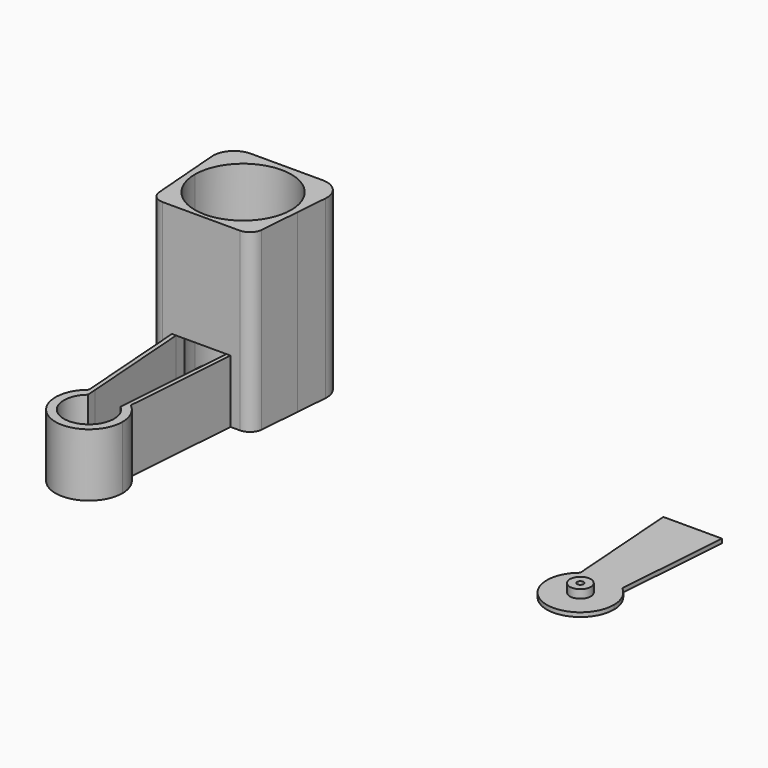
from build123d import *

# Parameters (mm, degrees)
F1_DEPTH  = 42
F2_DEPTH  = 15
F3_DEPTH  = 42
F4_DEPTH  = 15
F5_DEPTH  = 1
F0_R      = 2.5
F6_DEPTH  = 1
F0_R_2    = 1
F7_DEPTH  = 4
F8_DEPTH  = 1
F9_DEPTH  = 1
F0_R_3    = 0.75
F10_DEPTH = 3


with BuildPart() as f1:
    # F0 (on Top) → F1 (new body)
    with BuildSketch(Plane.XY):
        with BuildLine():
            Line((-12.9785589716, 24.8787840627), (-11.5, 24.8787840627))
            ThreePointArc((-11.5, 24.8787840627), (0, 36.3787840627), (11.5, 24.8787840627))
            Line((11.5, 24.8787840627), (12.9785589716, 24.8787840627))
            Line((12.9785589716, 24.8787840627), (13.5779219878, 32.533194811))
            ThreePointArc((13.5779219878, 32.533194811), (12.264120187, 36.318246043), (8.593180242, 37.923514843))
            Line((8.593180242, 37.923514843), (-8.593180242, 37.923514843))
            ThreePointArc((-8.593180242, 37.923514843), (-12.264120187, 36.318246043), (-13.5779219878, 32.533194811))
            Line((-13.5779219878, 32.533194811), (-12.9785589716, 24.8787840627))
        make_face()
        with BuildLine():
            ThreePointArc((11.5, 24.8787840627), (10.0894369384, 19.3603366119), (6.2037804754, 15.1956488363))
            Line((6.2037804754, 15.1956488363), (5.997311801, 12.3816961423))
            Line((5.997311801, 12.3816961423), (7, 12.3816961423))
            Line((7, 12.3816961423), (9.2257259033, 12.3816961423))
            ThreePointArc((9.2257259033, 12.3816961423), (11.2625646233, 13.1791321752), (12.2165709508, 15.1475041231))
            Line((12.2165709508, 15.1475041231), (12.9785589716, 24.8787840627))
            Line((12.9785589716, 24.8787840627), (11.5, 24.8787840627))
        make_face()
        with BuildLine():
            Line((-5.997311801, 12.3816961423), (-6.2037804754, 15.1956488363))
            ThreePointArc((-6.2037804754, 15.1956488363), (-10.0894369384, 19.3603366119), (-11.5, 24.8787840627))
            Line((-11.5, 24.8787840627), (-12.9785589716, 24.8787840627))
            Line((-12.9785589716, 24.8787840627), (-12.2165709508, 15.1475041231))
            ThreePointArc((-12.2165709508, 15.1475041231), (-11.2625646233, 13.1791321752), (-9.2257259033, 12.3816961423))
            Line((-9.2257259033, 12.3816961423), (-7, 12.3816961423))
            Line((-7, 12.3816961423), (-5.997311801, 12.3816961423))
        make_face()
    extrude(amount=F1_DEPTH)

    # F0 (on Top) → F2 (join)
    with BuildSketch(Plane.XY):
        with BuildLine():
            Line((-4.0454986584, -14.219481329), (-5.997311801, 12.3816961423))
            Line((-5.997311801, 12.3816961423), (-7, 12.3816961423))
            Line((-7, 12.3816961423), (-5, -14.8762179389))
            ThreePointArc((-5, -14.8762179389), (-4.5346540374, -14.5305473247), (-4.0454986584, -14.219481329))
        make_face()
        with BuildLine():
            Line((7, 12.3816961423), (5.997311801, 12.3816961423))
            Line((5.997311801, 12.3816961423), (4.0454986584, -14.219481329))
            ThreePointArc((4.0454986584, -14.219481329), (4.5346540374, -14.5305473247), (5, -14.8762179389))
            Line((5, -14.8762179389), (7, 12.3816961423))
        make_face()
        with BuildLine():
            Line((-3.8751972264, -16.5405122298), (-4.0454986584, -14.219481329))
            ThreePointArc((-4.0454986584, -14.219481329), (-4.5346540374, -14.5305473247), (-5, -14.8762179389))
            ThreePointArc((-5, -14.8762179389), (-3.4641016151, -28.3323184883), (8, -21.1212159373))
            ThreePointArc((8, -21.1212159373), (7.2111025509, -17.6571143222), (5, -14.8762179389))
            ThreePointArc((5, -14.8762179389), (4.5346540374, -14.5305473247), (4.0454986584, -14.219481329))
            Line((4.0454986584, -14.219481329), (3.8751972264, -16.5405122298))
            ThreePointArc((3.8751972264, -16.5405122298), (5.4429396175, -18.5964568754), (6, -21.1212159373))
            ThreePointArc((6, -21.1212159373), (-2.5247590619, -26.5641555548), (-3.8751972264, -16.5405122298))
        make_face()
    extrude(amount=F2_DEPTH)

    # F0 (on Top) → F3 (join)
    with BuildSketch(Plane.XY):
        with BuildLine():
            ThreePointArc((6.2037804754, 15.1956488363), (0, 13.3787840627), (-6.2037804754, 15.1956488363))
            Line((-6.2037804754, 15.1956488363), (-5.997311801, 12.3816961423))
            Line((-5.997311801, 12.3816961423), (5.997311801, 12.3816961423))
            Line((5.997311801, 12.3816961423), (6.2037804754, 15.1956488363))
        make_face()
    extrude(amount=F3_DEPTH)

    # F0 (on Top) → F4 (cut)
    with BuildSketch(Plane.XY):
        with BuildLine():
            ThreePointArc((6.2037804754, 15.1956488363), (0, 13.3787840627), (-6.2037804754, 15.1956488363))
            Line((-6.2037804754, 15.1956488363), (-5.997311801, 12.3816961423))
            Line((-5.997311801, 12.3816961423), (5.997311801, 12.3816961423))
            Line((5.997311801, 12.3816961423), (6.2037804754, 15.1956488363))
        make_face()
    extrude(amount=F4_DEPTH, mode=Mode.SUBTRACT)

    # F0 (on Top) → F5 (join)
    with BuildSketch(Plane.XY):
        with BuildLine():
            ThreePointArc((-11.5, 24.8787840627), (-10.0894369384, 19.3603366119), (-6.2037804754, 15.1956488363))
            ThreePointArc((-6.2037804754, 15.1956488363), (0, 13.3787840627), (6.2037804754, 15.1956488363))
            ThreePointArc((6.2037804754, 15.1956488363), (10.0894369384, 19.3603366119), (11.5, 24.8787840627))
            Line((11.5, 24.8787840627), (9.5, 24.8787840627))
            ThreePointArc((9.5, 24.8787840627), (0, 15.3787840627), (-9.5, 24.8787840627))
            Line((-9.5, 24.8787840627), (-11.5, 24.8787840627))
        make_face()
        with BuildLine():
            ThreePointArc((11.5, 24.8787840627), (0, 36.3787840627), (-11.5, 24.8787840627))
            Line((-11.5, 24.8787840627), (-9.5, 24.8787840627))
            ThreePointArc((-9.5, 24.8787840627), (0, 34.3787840627), (9.5, 24.8787840627))
            Line((9.5, 24.8787840627), (11.5, 24.8787840627))
        make_face()
        with BuildLine():
            Line((5.997311801, 12.3816961423), (-5.997311801, 12.3816961423))
            Line((-5.997311801, 12.3816961423), (-4.0454986584, -14.219481329))
            ThreePointArc((-4.0454986584, -14.219481329), (0, -13.1212159373), (4.0454986584, -14.219481329))
            Line((4.0454986584, -14.219481329), (5.997311801, 12.3816961423))
        make_face()
        with BuildLine():
            Line((0, 24.8787840627), (-9.5, 24.8787840627))
            ThreePointArc((-9.5, 24.8787840627), (0, 15.3787840627), (9.5, 24.8787840627))
            Line((9.5, 24.8787840627), (0, 24.8787840627))
        make_face()
        with BuildLine():
            ThreePointArc((9.5, 24.8787840627), (0, 34.3787840627), (-9.5, 24.8787840627))
            Line((-9.5, 24.8787840627), (0, 24.8787840627))
            Line((0, 24.8787840627), (9.5, 24.8787840627))
        make_face()
    extrude(amount=F5_DEPTH)

    # F0 (on Top) → F6 (join)
    with BuildSketch(Plane.XY):
        with BuildLine():
            Line((5.997311801, 12.3816961423), (-5.997311801, 12.3816961423))
            Line((-5.997311801, 12.3816961423), (-4.0454986584, -14.219481329))
            ThreePointArc((-4.0454986584, -14.219481329), (0, -13.1212159373), (4.0454986584, -14.219481329))
            Line((4.0454986584, -14.219481329), (5.997311801, 12.3816961423))
        make_face()
        with BuildLine():
            ThreePointArc((3.8751972264, -16.5405122298), (0, -15.1212159373), (-3.8751972264, -16.5405122298))
            ThreePointArc((-3.8751972264, -16.5405122298), (-2.5247590619, -26.5641555548), (6, -21.1212159373))
            ThreePointArc((6, -21.1212159373), (5.4429396175, -18.5964568754), (3.8751972264, -16.5405122298))
        make_face()
        with Locations((0, -21.1212159373)):
            Circle(F0_R, mode=Mode.SUBTRACT)
        with BuildLine():
            ThreePointArc((4.0454986584, -14.219481329), (0, -13.1212159373), (-4.0454986584, -14.219481329))
            Line((-4.0454986584, -14.219481329), (-3.8751972264, -16.5405122298))
            ThreePointArc((-3.8751972264, -16.5405122298), (0, -15.1212159373), (3.8751972264, -16.5405122298))
            Line((3.8751972264, -16.5405122298), (4.0454986584, -14.219481329))
        make_face()
        with BuildLine():
            ThreePointArc((6.2037804754, 15.1956488363), (0, 13.3787840627), (-6.2037804754, 15.1956488363))
            Line((-6.2037804754, 15.1956488363), (-5.997311801, 12.3816961423))
            Line((-5.997311801, 12.3816961423), (5.997311801, 12.3816961423))
            Line((5.997311801, 12.3816961423), (6.2037804754, 15.1956488363))
        make_face()
    extrude(amount=F6_DEPTH)

    # F0 (on Top) → F7 (join)
    with BuildSketch(Plane.XY):
        with Locations((0, -21.1212159373)):
            Circle(F0_R)
        with Locations((0, -21.1212159373)):
            Circle(F0_R_2, mode=Mode.SUBTRACT)
    extrude(amount=F7_DEPTH)

    # F0 (on Top) → F8 (join)
    with BuildSketch(Plane.XY):
        with Locations((0, -21.1212159373)):
            Circle(F0_R_2)
    extrude(amount=F8_DEPTH)


with BuildPart() as f5:
    # F0 (on Top) → F5, piece 2 (new body)
    with BuildSketch(Plane.XY):
        with BuildLine():
            Line((106.908822805, 32.923514843), (94.914199203, 32.923514843))
            Line((94.914199203, 32.923514843), (96.8660123455, 6.3223373718))
            ThreePointArc((96.8660123455, 6.3223373718), (100.911511004, 7.4206027634), (104.9570096624, 6.3223373718))
            Line((104.9570096624, 6.3223373718), (106.908822805, 32.923514843))
        make_face()
    extrude(amount=F5_DEPTH)

    # F0 (on Top) → F9 (join)
    with BuildSketch(Plane.XY):
        with BuildLine():
            Line((96.8660123455, 6.3223373718), (94.914199203, 32.923514843))
            Line((94.914199203, 32.923514843), (93.911511004, 32.923514843))
            Line((93.911511004, 32.923514843), (95.911511004, 5.6656007618))
            ThreePointArc((95.911511004, 5.6656007618), (96.3768569666, 6.011271376), (96.8660123455, 6.3223373718))
        make_face()
        with BuildLine():
            Line((107.911511004, 32.923514843), (106.908822805, 32.923514843))
            Line((106.908822805, 32.923514843), (104.9570096624, 6.3223373718))
            ThreePointArc((104.9570096624, 6.3223373718), (105.4461650413, 6.011271376), (105.911511004, 5.6656007618))
            Line((105.911511004, 5.6656007618), (107.911511004, 32.923514843))
        make_face()
        with BuildLine():
            Line((106.908822805, 32.923514843), (94.914199203, 32.923514843))
            Line((94.914199203, 32.923514843), (96.8660123455, 6.3223373718))
            ThreePointArc((96.8660123455, 6.3223373718), (100.911511004, 7.4206027634), (104.9570096624, 6.3223373718))
            Line((104.9570096624, 6.3223373718), (106.908822805, 32.923514843))
        make_face()
        with BuildLine():
            ThreePointArc((104.9570096624, 6.3223373718), (100.911511004, 7.4206027634), (96.8660123455, 6.3223373718))
            Line((96.8660123455, 6.3223373718), (97.0363137775, 4.0013064709))
            ThreePointArc((97.0363137775, 4.0013064709), (100.911511004, 5.4206027634), (104.7867082304, 4.0013064709))
            Line((104.7867082304, 4.0013064709), (104.9570096624, 6.3223373718))
        make_face()
        with BuildLine():
            Line((97.0363137775, 4.0013064709), (96.8660123455, 6.3223373718))
            ThreePointArc((96.8660123455, 6.3223373718), (96.3768569666, 6.011271376), (95.911511004, 5.6656007618))
            ThreePointArc((95.911511004, 5.6656007618), (97.4474093888, -7.7904997875), (108.911511004, -0.5793972366))
            ThreePointArc((108.911511004, -0.5793972366), (108.1226135549, 2.8847043785), (105.911511004, 5.6656007618))
            ThreePointArc((105.911511004, 5.6656007618), (105.4461650413, 6.011271376), (104.9570096624, 6.3223373718))
            Line((104.9570096624, 6.3223373718), (104.7867082304, 4.0013064709))
            ThreePointArc((104.7867082304, 4.0013064709), (106.3544506214, 1.9453618253), (106.911511004, -0.5793972366))
            ThreePointArc((106.911511004, -0.5793972366), (98.3867519421, -6.0223368541), (97.0363137775, 4.0013064709))
        make_face()
        with BuildLine():
            ThreePointArc((104.7867082304, 4.0013064709), (100.911511004, 5.4206027634), (97.0363137775, 4.0013064709))
            ThreePointArc((97.0363137775, 4.0013064709), (98.3867519421, -6.0223368541), (106.911511004, -0.5793972366))
            ThreePointArc((106.911511004, -0.5793972366), (106.3544506214, 1.9453618253), (104.7867082304, 4.0013064709))
        make_face()
        with Locations((100.911511004, -0.5793972366)):
            Circle(F0_R, mode=Mode.SUBTRACT)
    extrude(amount=F9_DEPTH)

    # F0 (on Top) → F10 (join)
    with BuildSketch(Plane.XY):
        with Locations((100.911511004, -0.5793972366)):
            Circle(F0_R)
        with Locations((100.911511004, -0.5793972366)):
            Circle(F0_R_3, mode=Mode.SUBTRACT)
    extrude(amount=F10_DEPTH)


solid = Compound([f1.part, f5.part])
